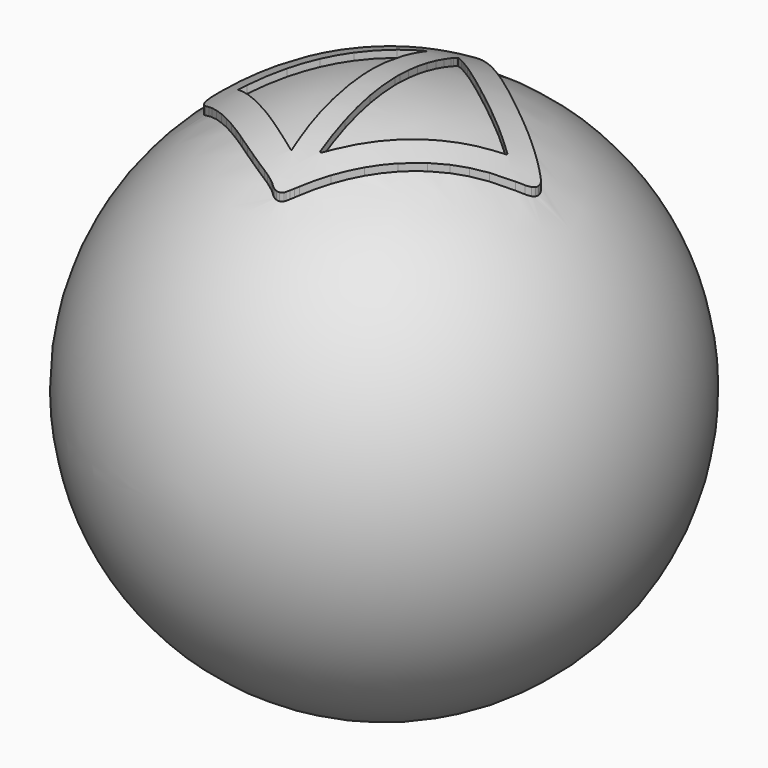
from build123d import *

# Parameters (mm, degrees)
F2_SCALE  = 33.3
F4_DEPTH  = 350
F5_SCALE  = 0.03
F8_SCALE  = 1.4
F9_R      = 2
F10_DEPTH = 25


# Not quite as in the source:
# - ends of sketch curves that miss each other by under 0.0002 mm in the source are joined


with BuildPart() as f1:
    # F0 (on Top) → F1 (revolve)
    with BuildSketch(Plane.XY):
        with BuildLine():
            ThreePointArc((0, 10), (-10, 0), (0, -10))
            Line((0, -10), (0, 10))
        make_face()
    revolve(axis=Axis((0, 0, 0), (0, 1, 0)))


with BuildPart() as f1_1:
    # F2: moved
    add(f1.part.scale(F2_SCALE))

    # F3 (on Top) → F4 (join)
    with BuildSketch(Plane.XY):
        with BuildLine():
            ThreePointArc((-27.5644771213, 174.7660485886), (-30.3473563419, 173.9827574855), (-32.9908772146, 172.8123904043))
            ThreePointArc((-32.9908772146, 172.8123904043), (-34.3738538233, 171.9806197142), (-35.6601525232, 171.0059904361))
            ThreePointArc((-35.6601525232, 171.0059904361), (-37.1492766243, 169.6725304876), (-38.5602295093, 168.2566144794))
            ThreePointArc((-38.5602295093, 168.2566144794), (-40.3746541592, 166.2518753997), (-42.1090761588, 164.1775331276))
            ThreePointArc((-42.1090761588, 164.1775331276), (-44.5506918075, 161.0964232622), (-46.951058847, 157.9830708836))
            ThreePointArc((-46.951058847, 157.9830708836), (-49.5923015521, 154.5246324845), (-52.2478739084, 151.0771849292))
            ThreePointArc((-52.2478739084, 151.0771849292), (-56.8787973877, 145.0965608582), (-61.5150183952, 139.1200425304))
            ThreePointArc((-61.5150183952, 139.1200425304), (-66.8935848678, 132.1995207862), (-72.2785574158, 125.2839825447))
            ThreePointArc((-72.2785574158, 125.2839825447), (-77.7591747353, 118.2587145355), (-83.2459858127, 111.2382828535))
            ThreePointArc((-83.2459858127, 111.2382828535), (-97.9548899032, 92.3117348205), (-112.5433909847, 73.2922259884))
            ThreePointArc((-112.5433909847, 73.2922259884), (-122.8213098488, 59.5666111302), (-132.8672873472, 45.6703362466))
            ThreePointArc((-132.8672873472, 45.6703362466), (-142.0054958632, 32.5434997776), (-150.8949014042, 19.2469152647))
            ThreePointArc((-150.8949014042, 19.2469152647), (-161.6628224285, 2.6266807331), (-172.2638067863, -14.1005261339))
            ThreePointArc((-172.2638067863, -14.1005261339), (-177.9652507412, -23.2246061066), (-183.6419658071, -32.3640921195))
            ThreePointArc((-183.6419658071, -32.3640921195), (-185.4779819962, -35.480094944), (-187.1752024704, -38.6738187632))
            ThreePointArc((-187.1752024704, -38.6738187632), (-188.0069611027, -40.6482808065), (-188.5642578347, -42.7170348348))
            ThreePointArc((-188.5642578347, -42.7170348348), (-188.8200276518, -44.7932407474), (-188.7719078351, -46.8845880802))
            ThreePointArc((-188.7719078351, -46.8845880802), (-188.2284646481, -49.8755647797), (-187.1928903456, -52.7336861591))
            ThreePointArc((-187.1928903456, -52.7336861591), (-185.6773295329, -55.4387578761), (-183.7543585872, -57.8711476169))
            ThreePointArc((-183.7543585872, -57.8711476169), (-180.9206408358, -60.6025266712), (-177.8009111204, -63.0020421759))
            ThreePointArc((-177.8009111204, -63.0020421759), (-173.0841977426, -66.0940819171), (-168.2494171091, -68.99804319))
            ThreePointArc((-168.2494171091, -68.99804319), (-164.7326054658, -71.0673020936), (-161.2606060503, -73.2109010796))
            ThreePointArc((-161.2606060503, -73.2109010796), (-155.3205732839, -76.9853725353), (-149.3980726695, -80.7872944877))
            ThreePointArc((-149.3980726695, -80.7872944877), (-142.5643392472, -85.2199131555), (-135.7520589508, -89.6854319253))
            ThreePointArc((-135.7520589508, -89.6854319253), (-128.8609026761, -94.2492886466), (-121.9908771125, -98.8448921673))
            ThreePointArc((-121.9908771125, -98.8448921673), (-115.1937594805, -103.4130878407), (-108.3953726327, -107.979394453))
            ThreePointArc((-108.3953726327, -107.979394453), (-101.8219291139, -112.3918080546), (-95.2471267583, -116.8021966395))
            ThreePointArc((-95.2471267583, -116.8021966395), (-89.633668075, -120.5652989004), (-84.0191330662, -124.3267950988))
            ThreePointArc((-84.0191330662, -124.3267950988), (-81.0066084709, -126.3409614023), (-77.9908770948, -128.3503231425))
            ThreePointArc((-77.9908770948, -128.3503231425), (-71.3907428485, -132.6671580135), (-64.7246630601, -136.8814450967))
            ThreePointArc((-64.7246630601, -136.8814450967), (-57.7917057233, -141.1222279239), (-50.7995379088, -145.2646578436))
            ThreePointArc((-50.7995379088, -145.2646578436), (-44.0339789011, -149.1428146532), (-37.2126589064, -152.9220318281))
            ThreePointArc((-37.2126589064, -152.9220318281), (-31.1352211996, -156.1486225351), (-24.9908769039, -159.2459068042))
            ThreePointArc((-24.9908769039, -159.2459068042), (-22.0647875277, -160.7093553163), (-19.1607513448, -162.2160916527))
            ThreePointArc((-19.1607513448, -162.2160916527), (-16.3844506703, -163.712381463), (-13.6333327625, -165.2544835844))
            ThreePointArc((-13.6333327625, -165.2544835844), (-11.3126581292, -166.6046323719), (-9.0131577807, -167.9905366424))
            ThreePointArc((-9.0131577807, -167.9905366424), (-7.8142374398, -168.798242432), (-6.6886001782, -169.7052922028))
            ThreePointArc((-6.6886001782, -169.7052922028), (-4.4818959837, -171.4622177718), (-2.1151628635, -172.9967877652))
            ThreePointArc((-2.1151628635, -172.9967877652), (0.044806521, -174.0346403894), (2.3408179707, -174.7208891361))
            ThreePointArc((2.3408179707, -174.7208891361), (4.5078832247, -174.9871164186), (6.6877359219, -174.8634604693))
            ThreePointArc((6.6877359219, -174.8634604693), (8.8702603881, -174.3549634488), (10.9391347329, -173.4937194834))
            ThreePointArc((10.9391347329, -173.4937194834), (11.7536316624, -172.9986403872), (12.4923881666, -172.3963551778))
            ThreePointArc((12.4923881666, -172.3963551778), (13.9513369599, -171.0040136558), (15.3845668839, -169.5852118849))
            ThreePointArc((15.3845668839, -169.5852118849), (17.0613110978, -167.8589589679), (18.7015785403, -166.0980094928))
            ThreePointArc((18.7015785403, -166.0980094928), (20.4161258533, -164.1854752905), (22.0975077694, -162.2437198038))
            ThreePointArc((22.0975077694, -162.2437198038), (32.4589246753, -150.2121745775), (42.9616115682, -138.3037486146))
            ThreePointArc((42.9616115682, -138.3037486146), (54.3124950484, -125.7091128301), (65.7849591362, -113.2251241264))
            ThreePointArc((65.7849591362, -113.2251241264), (77.1605475412, -101.0865215243), (88.6548334555, -89.0602554396))
            ThreePointArc((88.6548334555, -89.0602554396), (99.0738845848, -78.4122028178), (109.6374303708, -67.907482378))
            ThreePointArc((109.6374303708, -67.907482378), (117.8132781266, -59.9600695935), (126.0609977404, -52.0872697255))
            ThreePointArc((126.0609977404, -52.0872697255), (133.0217357647, -45.6050203508), (140.0825140569, -39.2318860641))
            ThreePointArc((140.0825140569, -39.2318860641), (147.6111066148, -32.6384047559), (155.233807517, -26.1539516167))
            ThreePointArc((155.233807517, -26.1539516167), (165.2976247474, -17.772772334), (175.4159893499, -9.4575284286))
            ThreePointArc((175.4159893499, -9.4575284286), (179.0498902818, -6.3857980092), (182.5764210169, -3.191374018))
            ThreePointArc((182.5764210169, -3.191374018), (184.7149177076, -0.93984506), (186.57853976, 1.5439954959))
            ThreePointArc((186.57853976, 1.5439954959), (187.7124463985, 3.6316819013), (188.4626315423, 5.8858781087))
            ThreePointArc((188.4626315423, 5.8858781087), (188.8125193502, 8.2525070903), (188.7505621476, 10.6440580166))
            ThreePointArc((188.7505621476, 10.6440580166), (188.4220099851, 12.488259503), (187.8605060143, 14.2753630055))
            ThreePointArc((187.8605060143, 14.2753630055), (187.0883931914, 15.9219493763), (186.0941301166, 17.4447250883))
            ThreePointArc((186.0941301166, 17.4447250883), (184.4802402167, 19.4106547715), (182.718200679, 21.2449767051))
            ThreePointArc((182.718200679, 21.2449767051), (179.3031969136, 24.4869807241), (175.8424080848, 27.6800640932))
            ThreePointArc((175.8424080848, 27.6800640932), (171.1087115633, 31.8758294115), (166.2688138142, 35.9486317733))
            ThreePointArc((166.2688138142, 35.9486317733), (160.2263855326, 40.8320029345), (154.1162909541, 45.6304399407))
            ThreePointArc((154.1162909541, 45.6304399407), (146.9258592718, 51.1265517296), (139.6687932957, 56.5343744019))
            ThreePointArc((139.6687932957, 56.5343744019), (131.3641290621, 62.5909319775), (123.0091231922, 68.5778522706))
            ThreePointArc((123.0091231922, 68.5778522706), (114.4026630281, 74.7230411226), (105.8269742542, 80.9110993504))
            ThreePointArc((105.8269742542, 80.9110993504), (98.4993369127, 86.2705249451), (91.2140617183, 91.6873946242))
            ThreePointArc((91.2140617183, 91.6873946242), (83.1809645054, 97.7514885169), (75.1885660827, 103.8691231073))
            ThreePointArc((75.1885660827, 103.8691231073), (64.0879146767, 112.4474094878), (53.0091226993, 121.0539086139))
            ThreePointArc((53.0091226993, 121.0539086139), (42.988531858, 128.8341320836), (32.9440871045, 136.5835351358))
            ThreePointArc((32.9440871045, 136.5835351358), (25.3550420973, 142.3774754358), (17.7252818072, 148.1176937418))
            ThreePointArc((17.7252818072, 148.1176937418), (11.2853128443, 152.8827575875), (4.8031713399, 157.5902914725))
            ThreePointArc((4.8031713399, 157.5902914725), (-1.5070977953, 162.0832534986), (-7.8613066131, 166.5138555608))
            ThreePointArc((-7.8613066131, 166.5138555608), (-12.2927406943, 169.4628507588), (-16.8207034637, 172.2613742207))
            ThreePointArc((-16.8207034637, 172.2613742207), (-19.6428893356, 173.6736856403), (-22.6401269856, 174.6615740576))
            ThreePointArc((-22.6401269856, 174.6615740576), (-25.0964170735, 174.9911947522), (-27.5644771213, 174.7660485886))
        make_face()
        with BuildLine():
            ThreePointArc((-36.2158216276, 87.8874170202), (-35.875365993, 81.4653158167), (-35.5492196272, 75.0424720185))
            ThreePointArc((-35.5492196272, 75.0424720185), (-34.7694743462, 59.800442664), (-33.9442495261, 44.5608079707))
            ThreePointArc((-33.9442495261, 44.5608079707), (-33.3232527433, 34.2553037971), (-32.6075567606, 23.9559430177))
            ThreePointArc((-32.6075567606, 23.9559430177), (-31.840545287, 14.2798029253), (-30.9743380128, 4.6120379988))
            ThreePointArc((-30.9743380128, 4.6120379988), (-29.7333556554, -8.1756084738), (-28.4347134709, -20.9575280489))
            ThreePointArc((-28.4347134709, -20.9575280489), (-26.8711179752, -35.7491375424), (-25.2539878727, -50.5349899858))
            ThreePointArc((-25.2539878727, -50.5349899858), (-23.8860532006, -62.4661424027), (-22.4368286951, -74.3876939619))
            ThreePointArc((-22.4368286951, -74.3876939619), (-21.1443944217, -84.3882722353), (-19.7690809539, -94.3777899935))
            ThreePointArc((-19.7690809539, -94.3777899935), (-18.4668744547, -103.172368085), (-17.0585632073, -111.9505800345))
            ThreePointArc((-17.0585632073, -111.9505800345), (-16.5037009331, -115.3123264447), (-15.9591894627, -118.6757649139))
            ThreePointArc((-15.9591894627, -118.6757649139), (-15.5095526909, -121.526486539), (-15.0742946729, -124.3794389509))
            ThreePointArc((-15.0742946729, -124.3794389509), (-14.6946148385, -126.9163416525), (-14.3165330004, -129.453483))
            ThreePointArc((-14.3165330004, -129.453483), (-14.3277996451, -129.5847246485), (-14.3968909938, -129.6968750062))
            ThreePointArc((-14.3968909938, -129.6968750062), (-14.7688654636, -129.8774224631), (-15.1728080327, -129.7891460536))
            ThreePointArc((-15.1728080327, -129.7891460536), (-21.7670796052, -125.7536255332), (-28.3572800281, -121.7114600458))
            ThreePointArc((-28.3572800281, -121.7114600458), (-35.1022240881, -117.5330113861), (-41.8140330509, -113.3015430801))
            ThreePointArc((-41.8140330509, -113.3015430801), (-48.4198165665, -109.0625816585), (-54.9908768565, -104.7699907823))
            ThreePointArc((-54.9908768565, -104.7699907823), (-69.1326880806, -95.4655679062), (-83.2893122183, -86.1836983336))
            ThreePointArc((-83.2893122183, -86.1836983336), (-95.6925842251, -78.0865854409), (-108.1150440078, -70.018941012))
            ThreePointArc((-108.1150440078, -70.018941012), (-118.1965570891, -63.506309534), (-128.2941642625, -57.0186594098))
            ThreePointArc((-128.2941642625, -57.0186594098), (-134.2286420334, -53.2625289121), (-140.2045128346, -49.5726087287))
            Line((-140.2045128346, -49.5726087287), (-152.918148, -41.819607))
            Line((-152.918148, -41.819607), (-147.804557, -33.638567))
            ThreePointArc((-147.804557, -33.638567), (-136.6192352895, -15.9410715729), (-125.2575372338, 1.6437111527))
            ThreePointArc((-125.2575372338, 1.6437111527), (-115.7195505944, 15.9638832924), (-105.9269792984, 30.1111822105))
            ThreePointArc((-105.9269792984, 30.1111822105), (-95.6789766631, 44.3730449468), (-85.1852609553, 58.4550979661))
            ThreePointArc((-85.1852609553, 58.4550979661), (-71.7276729444, 76.0311792744), (-58.1167072705, 93.4887542128))
            Line((-58.1167072705, 93.4887542128), (-38.490877, 118.435036))
            Line((-38.490877, 118.435036), (-37.827045, 112.988754))
            ThreePointArc((-37.827045, 112.988754), (-37.6349122305, 111.2002153631), (-37.4939133421, 109.406920978))
            ThreePointArc((-37.4939133421, 109.406920978), (-37.1838137595, 104.5015043667), (-36.8841044388, 99.5954419737))
            ThreePointArc((-36.8841044388, 99.5954419737), (-36.5413640971, 93.7419203165), (-36.2158216276, 87.8874170202))
        make_face(mode=Mode.SUBTRACT)
        with BuildLine():
            ThreePointArc((-5.7300527742, 126.8047383051), (-1.6039551452, 123.737072354), (2.5091232309, 120.6519723065))
            ThreePointArc((2.5091232309, 120.6519723065), (4.6974058159, 118.9933789275), (6.8760225175, 117.3221093748))
            ThreePointArc((6.8760225175, 117.3221093748), (10.5304128715, 114.4979281794), (14.1809980431, 111.6688300555))
            ThreePointArc((14.1809980431, 111.6688300555), (18.3797485741, 108.4057193009), (22.5739659539, 105.136783941))
            ThreePointArc((22.5739659539, 105.136783941), (26.7937892984, 101.8385585234), (31.0091230551, 98.5345970701))
            ThreePointArc((31.0091230551, 98.5345970701), (40.4693535888, 91.1402914937), (49.9595121253, 83.7844361623))
            ThreePointArc((49.9595121253, 83.7844361623), (57.4315287562, 78.0665343861), (64.9508813171, 72.4110264252))
            ThreePointArc((64.9508813171, 72.4110264252), (72.3282827924, 66.9597051443), (79.7525830906, 61.572431126))
            ThreePointArc((79.7525830906, 61.572431126), (88.8653105522, 55.0529984048), (98.0091228072, 48.5772357263))
            ThreePointArc((98.0091228072, 48.5772357263), (108.9442542056, 40.8139536921), (119.8241321574, 32.9734242169))
            ThreePointArc((119.8241321574, 32.9734242169), (127.8977462244, 27.0091299624), (135.871650036, 20.9121710462))
            ThreePointArc((135.871650036, 20.9121710462), (142.0823685212, 16.0468412877), (148.2592019731, 11.1385639664))
            ThreePointArc((148.2592019731, 11.1385639664), (148.8726091299, 10.1945493949), (148.8016497413, 9.0709851042))
            ThreePointArc((148.8016497413, 9.0709851042), (148.6637703672, 8.8174288561), (148.4715711567, 8.6021128237))
            ThreePointArc((148.4715711567, 8.6021128237), (147.1398313123, 7.4218446143), (145.8044277187, 6.2457233203))
            ThreePointArc((145.8044277187, 6.2457233203), (144.2436997983, 4.8873844546), (142.6712590306, 3.5426219639))
            ThreePointArc((142.6712590306, 3.5426219639), (140.8445228181, 2.0028772411), (139.0091227133, 0.4734703461))
            ThreePointArc((139.0091227133, 0.4734703461), (126.2763575386, -10.359906706), (113.8314791775, -21.5228081928))
            ThreePointArc((113.8314791775, -21.5228081928), (99.6282848414, -34.8226415944), (85.6485942113, -48.3572102147))
            ThreePointArc((85.6485942113, -48.3572102147), (70.6746216813, -63.3289912655), (55.9352563791, -78.5317933619))
            ThreePointArc((55.9352563791, -78.5317933619), (40.8899252231, -94.5154279338), (26.0691810409, -110.7075280369))
            ThreePointArc((26.0691810409, -110.7075280369), (24.2770648812, -112.6786188957), (22.470623706, -114.6365897267))
            ThreePointArc((22.470623706, -114.6365897267), (20.9060909697, -116.3006649337), (19.3224758969, -117.9465908997))
            ThreePointArc((19.3224758969, -117.9465908997), (17.9457723446, -119.3560269346), (16.5640628229, -120.7605558252))
            ThreePointArc((16.5640628229, -120.7605558252), (16.3481902472, -120.9063038689), (16.092809, -120.957528))
            ThreePointArc((16.092809, -120.957528), (14.9267971459, -120.5172937175), (14.3426865235, -119.4162920607))
            ThreePointArc((14.3426865235, -119.4162920607), (11.3949337842, -96.1849115038), (8.4725977277, -72.9503200341))
            ThreePointArc((8.4725977277, -72.9503200341), (5.6315941027, -49.4602175208), (2.9884735346, -25.9470269422))
            ThreePointArc((2.9884735346, -25.9470269422), (0.6666566092, -3.4629650138), (-1.4379052435, 19.0424719784))
            ThreePointArc((-1.4379052435, 19.0424719784), (-1.8240663076, 23.6496777434), (-2.1660653276, 28.2603720466))
            ThreePointArc((-2.1660653276, 28.2603720466), (-2.6522225322, 35.4117064449), (-3.118768656, 42.564347022))
            ThreePointArc((-3.118768656, 42.564347022), (-3.6230131674, 50.6367360275), (-4.1049758324, 58.7104860098))
            ThreePointArc((-4.1049758324, 58.7104860098), (-4.5548891541, 66.6258368816), (-4.9816087242, 74.5424720145))
            ThreePointArc((-4.9816087242, 74.5424720145), (-5.3825722179, 82.1072595728), (-5.792143451, 89.6715859753))
            ThreePointArc((-5.792143451, 89.6715859753), (-6.1809641905, 96.685892654), (-6.5798007046, 103.6996369594))
            ThreePointArc((-6.5798007046, 103.6996369594), (-6.922087944, 109.5855076818), (-7.2711085488, 115.4709829671))
            ThreePointArc((-7.2711085488, 115.4709829671), (-7.4338536406, 117.9560812693), (-7.6243817889, 120.4392040174))
            ThreePointArc((-7.6243817889, 120.4392040174), (-7.8461004292, 123.4588335688), (-8.0141838332, 126.4819230078))
            ThreePointArc((-8.0141838332, 126.4819230078), (-7.8067440215, 127.0459132728), (-7.258069013, 127.2910096179))
            ThreePointArc((-7.258069013, 127.2910096179), (-6.4536885388, 127.1747365122), (-5.7300527742, 126.8047383051))
        make_face(mode=Mode.SUBTRACT)
    extrude(amount=F4_DEPTH)


with BuildPart() as f1_2:
    # F5: moved
    add(f1_1.part.scale(F5_SCALE))

    # F6 (on Top) → F7 (revolve, cut)
    with BuildSketch(Plane.XY):
        with BuildLine():
            Line((0, 10.25), (0, 15))
            ThreePointArc((0, 15), (-15, 0), (0, -15))
            Line((0, -15), (0, -10.25))
            ThreePointArc((0, -10.25), (-10.25, 0), (0, 10.25))
        make_face()
        with BuildLine():
            Line((0, -7), (0, 7))
            ThreePointArc((0, 7), (-7, 0), (0, -7))
        make_face()
    revolve(axis=Axis((0, 0, 0), (0, -1, 0)), mode=Mode.SUBTRACT)


with BuildPart() as f1_3:
    # F8: moved
    add(f1_2.part.scale(F8_SCALE))

    # F9 (on Front) → F10 (cut)
    with BuildSketch(Plane.XZ):
        with Locations((0, -5.1200183504)):
            Circle(F9_R)
    extrude(amount=-F10_DEPTH, mode=Mode.SUBTRACT)


solid = f1_3.part
